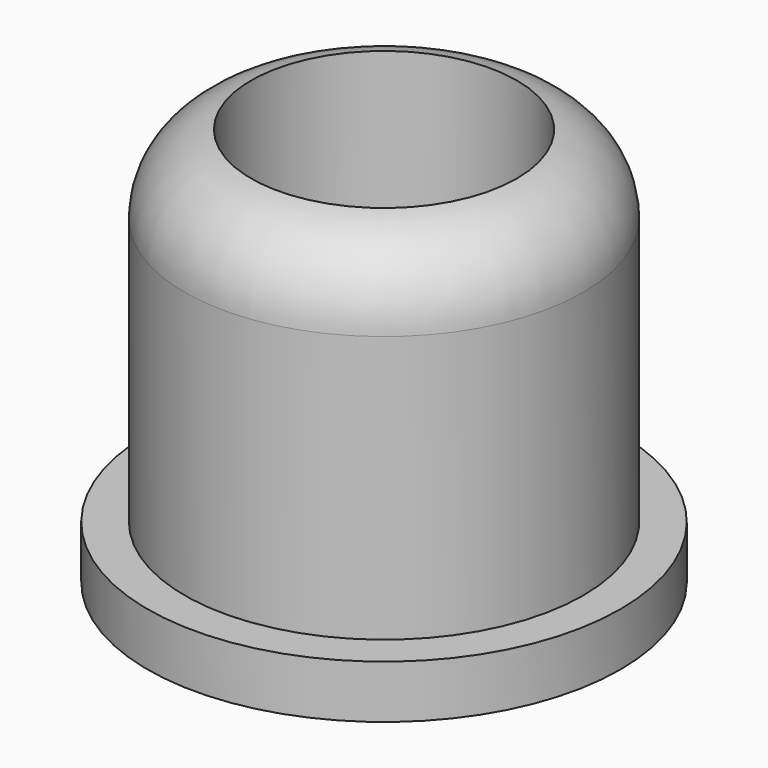
from build123d import *

# Parameters (mm, degrees)
F0_R     = 7.5
F1_DEPTH = 15
F2_R     = 8.8984666771
F2_R_2   = 7.5
F3_DEPTH = 2
F4_T     = 2.5


# Not quite as in the source:
# - a fillet or chamfer that OpenCascade refuses, or shapes differently, is made with other operations: its cross-section is extruded or revolved along the edge and cut away or added
# - a shell that OpenCascade refuses in one call is made with other operations: the cavity is built on its own and cut out


with BuildPart() as f1:
    # F0 (on Top) → F1 (new body)
    with BuildSketch(Plane.XY):
        Circle(F0_R)
    extrude(amount=F1_DEPTH)

    # F2 (on face) → F3 (join)
    with BuildSketch(Plane.XY):
        Circle(F2_R)
        Circle(F2_R_2, mode=Mode.SUBTRACT)
    extrude(amount=F3_DEPTH)

    # F4: shell of thickness 2.5, made by hand


with BuildPart() as f4_core1:
    # F4_t2: copy of F1
    add(f1.part)

    # the walls: a layer under each face that stays
    f4_faces = [f4_core1.faces().sort_by_distance(p)[0] for p in [
        (-7.5, 0, 8.5),
        (-5.9323111181, -5.9323111181, 2),
        (-8.8984666771, 0, 1),
    ]]
    thicken(f4_faces, amount=-F4_T, mode=Mode.SUBTRACT)

    # F4_s3 → F4_t4 (revolve, cut)
    with BuildSketch(Plane.XZ):
        Polygon((7.525, 2.025), (5, 2), (5, -0.5), (7.5, -0.5), align=None)
    revolve(axis=Axis((0, 0, 2), (0, 0, 1)), mode=Mode.SUBTRACT)


with BuildPart() as f1_1:
    add(f1.part)

    # what is left inside the walls is the cavity
    f4_cavity = [f4_core1.part.solids().sort_by_distance(p)[0] for p in [
        (-4.975, 0, 10),
    ]]
    add(f4_cavity, mode=Mode.SUBTRACT)

    # F5: fillet of radius 3 on 1 edges, made by hand

    # F5_s1 → F5_t2 (revolve, cut)
    with BuildSketch(Plane.XZ):
        with BuildLine():
            ThreePointArc((7.5, 12.0419601084), (6.7912878475, 13.9784517816), (5, 15))
            Line((5, 15), (7.5, 15))
            Line((7.5, 15), (7.5, 12.0419601084))
        make_face()
    revolve(axis=Axis((0, 0, 15), (0, 0, 1)), mode=Mode.SUBTRACT)


solid = f1_1.part
